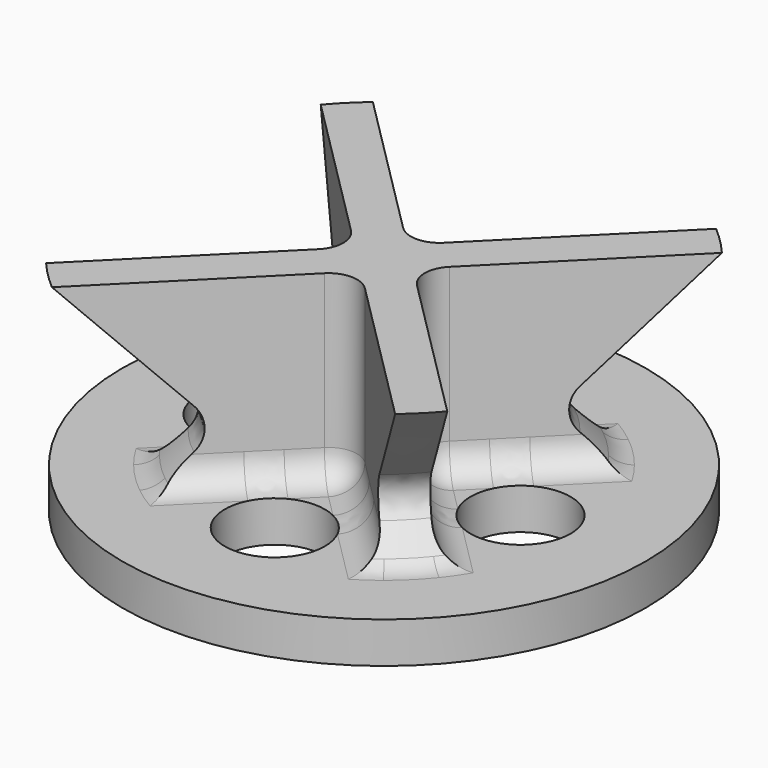
from build123d import *

# Parameters (mm, degrees)
F1_R      = 11.5
F3_DEPTH  = 1.8
F2_R      = 2.2
F4_DEPTH  = 25
F6_DEPTH  = 8
F11_F1_R  = 1.2553910524
F11_F2_R  = 1.2553910524
F11_F3_R  = 1.2553910524
F11_F4_R  = 1.2553910524
F11_F5_R  = 1.2553910524
F11_F6_R  = 1.2553910524
F11_F7_R  = 1.2553910524
F11_F8_R  = 1.2553910524
F11_F9_R  = 1.2553910524
F11_F10_R = 1.2553910524
F11_F11_R = 1.2553910524
F11_F12_R = 1.2553910524
F11_F13_R = 1.2553910524
F11_F14_R = 1.2553910524
F11_F15_R = 1.2553910524
F11_F16_R = 1.2553910524
F12_R     = 2
F13_DEPTH = 0.5


# Not quite as in the source:
# - a feature names something its author has since deleted; it is built from what else it names


with BuildPart() as f3:
    # F1 (on Top) → F3 (new body)
    with BuildSketch(Plane.XY):
        Circle(F1_R)
    extrude(amount=F3_DEPTH)

    # F2 (on face) → F4 (cut)
    with BuildSketch(Plane.XY):
        with Locations((0, 6)):
            Circle(F2_R)
        with Locations((-6, 0)):
            Circle(F2_R)
        with Locations((0, -6)):
            Circle(F2_R)
        with Locations((6, 0)):
            Circle(F2_R)
    extrude(amount=F4_DEPTH, mode=Mode.SUBTRACT)

    # F5 (on face) → F6 (join)
    with BuildSketch(Plane.XY.offset(1.8)):
        with BuildLine():
            Line((11.2429978209, -9.9702056147), (8.7431833829, -7.4703911767))
            ThreePointArc((8.7431833829, -7.4703911767), (8.1317279836, -8.1317279836), (7.4703911767, -8.7431833829))
            Line((7.4703911767, -8.7431833829), (9.9702056147, -11.2429978209))
            Line((9.9702056147, -11.2429978209), (11.2429978209, -9.9702056147))
        make_face()
        with BuildLine():
            Line((8.7431833829, -7.4703911767), (1.2727922061, 0))
            Line((1.2727922061, 0), (0, -1.2727922061))
            Line((0, -1.2727922061), (7.4703911767, -8.7431833829))
            ThreePointArc((7.4703911767, -8.7431833829), (8.1317279836, -8.1317279836), (8.7431833829, -7.4703911767))
        make_face()
        with BuildLine():
            ThreePointArc((-7.4703911767, -8.7431833829), (-8.1317279836, -8.1317279836), (-8.7431833829, -7.4703911767))
            Line((-8.7431833829, -7.4703911767), (-11.2429978209, -9.9702056147))
            Line((-11.2429978209, -9.9702056147), (-9.9702056147, -11.2429978209))
            Line((-9.9702056147, -11.2429978209), (-7.4703911767, -8.7431833829))
        make_face()
        with BuildLine():
            Line((0, -1.2727922061), (-1.2727922061, 0))
            Line((-1.2727922061, 0), (-8.7431833829, -7.4703911767))
            ThreePointArc((-8.7431833829, -7.4703911767), (-8.1317279836, -8.1317279836), (-7.4703911767, -8.7431833829))
            Line((-7.4703911767, -8.7431833829), (0, -1.2727922061))
        make_face()
        Polygon((1.2727922061, 0), (0, 1.2727922061), (-1.2727922061, 0), (0, -1.2727922061), align=None)
        with BuildLine():
            Line((-1.2727922061, 0), (0, 1.2727922061))
            Line((0, 1.2727922061), (-7.4703911767, 8.7431833829))
            ThreePointArc((-7.4703911767, 8.7431833829), (-8.1317279836, 8.1317279836), (-8.7431833829, 7.4703911767))
            Line((-8.7431833829, 7.4703911767), (-1.2727922061, 0))
        make_face()
        with BuildLine():
            ThreePointArc((-8.7431833829, 7.4703911767), (-8.1317279836, 8.1317279836), (-7.4703911767, 8.7431833829))
            Line((-7.4703911767, 8.7431833829), (-9.9702056147, 11.2429978209))
            Line((-9.9702056147, 11.2429978209), (-11.2429978209, 9.9702056147))
            Line((-11.2429978209, 9.9702056147), (-8.7431833829, 7.4703911767))
        make_face()
        with BuildLine():
            ThreePointArc((8.7431833829, 7.4703911767), (8.1317279836, 8.1317279836), (7.4703911767, 8.7431833829))
            Line((7.4703911767, 8.7431833829), (0, 1.2727922061))
            Line((0, 1.2727922061), (1.2727922061, 0))
            Line((1.2727922061, 0), (8.7431833829, 7.4703911767))
        make_face()
        with BuildLine():
            Line((11.2429978209, 9.9702056147), (9.9702056147, 11.2429978209))
            Line((9.9702056147, 11.2429978209), (7.4703911767, 8.7431833829))
            ThreePointArc((7.4703911767, 8.7431833829), (8.1317279836, 8.1317279836), (8.7431833829, 7.4703911767))
            Line((8.7431833829, 7.4703911767), (11.2429978209, 9.9702056147))
        make_face()
    extrude(amount=F6_DEPTH)

    # F9 (on mid) → F10 (revolve, cut)
    with BuildSketch(Plane(origin=(0, 0, 0), x_dir=(0.7071067812, -0.7071067812, 0), z_dir=(-0.7071067812, -0.7071067812, 0))):
        Polygon((-26.3970314711, 24.5940629423), (-26.3970314711, 1.8), (-8.0732320203, 1.8), (-5.8381002746, 4.0351317457), align=None)
    revolve(axis=Axis((0, 0, 20.9964681417), (0, 0, 1)), mode=Mode.SUBTRACT)

    # F11: fillet of radius 1.2553910524 on 20 edges, made by hand

    # F11_f1
    f11_f1_edges = [f3.edges().sort_by_distance(p)[0] for p in [
        (1.2727922061, 0, 5.8),
    ]]
    fillet(f11_f1_edges, radius=F11_F1_R)

    # F11_f2
    f11_f2_edges = [f3.edges().sort_by_distance(p)[0] for p in [
        (0, 1.2727922061, 5.8),
    ]]
    fillet(f11_f2_edges, radius=F11_F2_R)

    # F11_f3
    f11_f3_edges = [f3.edges().sort_by_distance(p)[0] for p in [
        (-1.2727922061, 0, 5.8),
    ]]
    fillet(f11_f3_edges, radius=F11_F3_R)

    # F11_f4
    f11_f4_edges = [f3.edges().sort_by_distance(p)[0] for p in [
        (0, -1.2727922061, 5.8),
    ]]
    fillet(f11_f4_edges, radius=F11_F4_R)

    # F11_f5
    f11_f5_edges = [f3.edges().sort_by_distance(p)[0] for p in [
        (-4.2349687388, 2.9621765326, 1.8),
    ]]
    fillet(f11_f5_edges, radius=F11_F5_R)

    # F11_f6
    f11_f6_edges = [f3.edges().sort_by_distance(p)[0] for p in [
        (-2.9621765326, 4.2349687388, 1.8),
    ]]
    fillet(f11_f6_edges, radius=F11_F6_R)

    # F11_f7
    f11_f7_edges = [f3.edges().sort_by_distance(p)[0] for p in [
        (4.2349687388, 2.9621765326, 1.8),
    ]]
    fillet(f11_f7_edges, radius=F11_F7_R)

    # F11_f8
    f11_f8_edges = [f3.edges().sort_by_distance(p)[0] for p in [
        (-2.9621765326, -4.2349687388, 1.8),
    ]]
    fillet(f11_f8_edges, radius=F11_F8_R)

    # F11_f9
    f11_f9_edges = [f3.edges().sort_by_distance(p)[0] for p in [
        (-4.1281602934, 4.1281602934, 4.0351317457),
    ]]
    fillet(f11_f9_edges, radius=F11_F9_R)

    # F11_f10
    f11_f10_edges = [f3.edges().sort_by_distance(p)[0] for p in [
        (4.1281602934, 4.1281602934, 4.0351317457),
    ]]
    fillet(f11_f10_edges, radius=F11_F10_R)

    # F11_f11
    f11_f11_edges = [f3.edges().sort_by_distance(p)[0] for p in [
        (-4.1281602934, -4.1281602934, 4.0351317457),
    ]]
    fillet(f11_f11_edges, radius=F11_F11_R)

    # F11_f12
    f11_f12_edges = [f3.edges().sort_by_distance(p)[0] for p in [
        (4.1281602934, -4.1281602934, 4.0351317457),
    ]]
    fillet(f11_f12_edges, radius=F11_F12_R)

    # F11_f13
    f11_f13_edges = [f3.edges().sort_by_distance(p)[0] for p in [
        (5.7086371076, -5.7086371076, 1.8),
    ]]
    fillet(f11_f13_edges, radius=F11_F13_R)

    # F11_f14
    f11_f14_edges = [f3.edges().sort_by_distance(p)[0] for p in [
        (5.7086371076, 5.7086371076, 1.8),
    ]]
    fillet(f11_f14_edges, radius=F11_F14_R)

    # F11_f15
    f11_f15_edges = [f3.edges().sort_by_distance(p)[0] for p in [
        (-5.7086371076, -5.7086371076, 1.8),
    ]]
    fillet(f11_f15_edges, radius=F11_F15_R)

    # F11_f16
    f11_f16_edges = [f3.edges().sort_by_distance(p)[0] for p in [
        (-5.7086371076, 5.7086371076, 1.8),
    ]]
    fillet(f11_f16_edges, radius=F11_F16_R)

    # F12 (on face) → F13 (cut)
    with BuildSketch(Plane.XY.offset(1.8)):
        with Locations((0, 6)):
            Circle(F12_R)
        with Locations((-6, 0)):
            Circle(F12_R)
        with Locations((0, -6)):
            Circle(F12_R)
        with Locations((6, 0)):
            Circle(F12_R)
    extrude(amount=-F13_DEPTH, mode=Mode.SUBTRACT)


solid = f3.part
